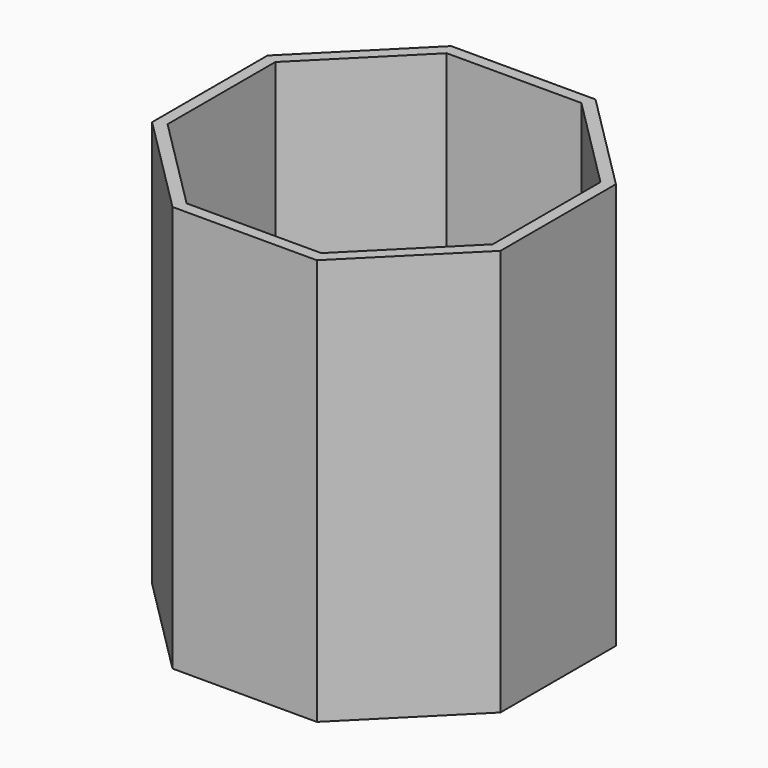
from build123d import *

# Parameters (mm, degrees)
F1_DEPTH     = 88.9
F3_DEPTH     = 82.55
F4_TEXT_SIZE = 43.8376020178
F5_DEPTH     = 3.175


# Not quite as in the source:
# - Text() gives the source's letters only with a copy of the font that has no kerning and outlines rounded to 1/6400 em; it was checked with that copy


with BuildPart() as f1:
    # F0 (on Top) → F1 (new body)
    with BuildSketch(Plane.XY):
        Polygon((38.1, -15.7815367264), (38.1, 15.7815367264), (15.7815367264, 38.1), (-15.7815367264, 38.1), (-38.1, 15.7815367264), (-38.1, -15.7815367264), (-15.7815367264, -38.1), (15.7815367264, -38.1), align=None)
    extrude(amount=F1_DEPTH)

    # F2 (on face) → F3 (cut)
    with BuildSketch(Plane.XY.offset(88.9)):
        Polygon((35.56, -14.729434278), (35.56, 14.729434278), (14.729434278, 35.56), (-14.729434278, 35.56), (-35.56, 14.729434278), (-35.56, -14.729434278), (-14.729434278, -35.56), (14.729434278, -35.56), align=None)
    extrude(amount=-F3_DEPTH, mode=Mode.SUBTRACT)

    # F4 (on face) → F5 (cut)
    with BuildSketch(Plane(origin=(0, 0, 0), x_dir=(1, 0, 0), z_dir=(0, 0, -1))):
        with Locations((-34.0966591478, -15.748)):
            Text('Lial', F4_TEXT_SIZE, font='Open Sans', text_align=(TextAlign.LEFT, TextAlign.BOTTOM))
    extrude(amount=-F5_DEPTH, mode=Mode.SUBTRACT)


solid = f1.part
